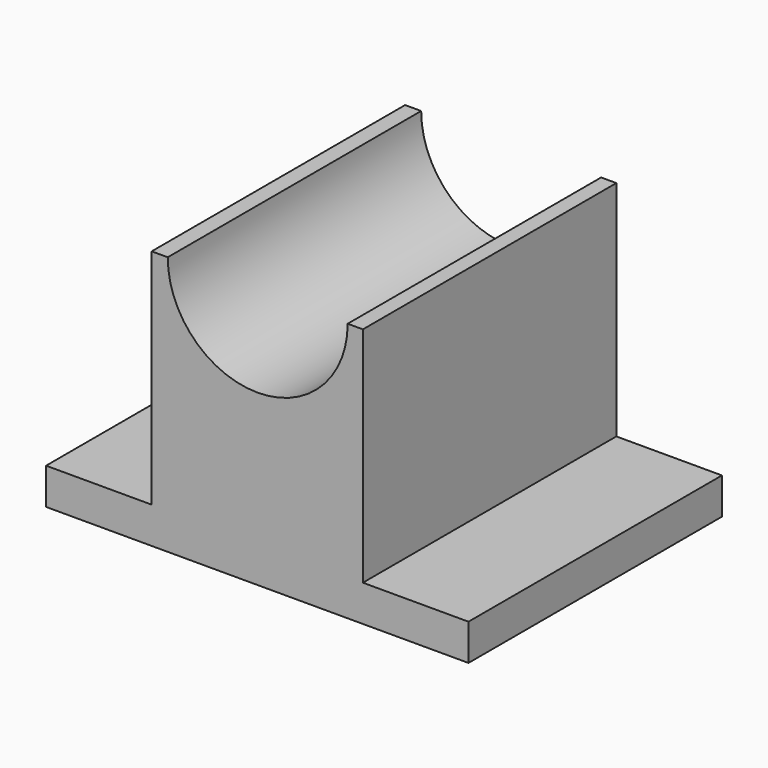
from build123d import *

# Parameters (mm, degrees)
F1_DEPTH = 114.3
F2_DEPTH = 114.3


# Not quite as in the source:
# - a feature names something its author has since deleted; it is built from what else it names


with BuildPart() as f1:
    # F0 (on Front) → F1 (new body)
    with BuildSketch(Plane.XZ):
        with BuildLine():
            Line((-32.3088020086, 46.7868000269), (-38.1029994101, 46.7868000269))
            Line((-38.1029994101, 46.7868000269), (-38.1029994101, -33.6804017425))
            Line((-38.1029994101, -33.6804017425), (-76.2000009418, -33.6804017425))
            Line((-76.2000009418, -33.6804017425), (-76.2000009418, -46.7868000269))
            Line((-76.2000009418, -46.7868000269), (-38.1029994101, -46.7868000269))
            Line((-38.1029994101, -46.7868000269), (38.1029994101, -46.7868000269))
            Line((38.1029994101, -46.7868000269), (76.2000009418, -46.7868000269))
            Line((76.2000009418, -46.7868000269), (76.2000009418, -33.6804017425))
            Line((76.2000009418, -33.6804017425), (38.1029994101, -33.6804017425))
            Line((38.1029994101, -33.6804017425), (38.1029994101, 46.7868000269))
            Line((38.1029994101, 46.7868000269), (32.6135978103, 46.7868000269))
            ThreePointArc((32.6135978103, 46.7868000269), (0.1523979008, 14.3256001174), (-32.3088020086, 46.7868000269))
        make_face()
    extrude(amount=F1_DEPTH)


with BuildPart() as f2:
    # F0 (on Front) → F2 (new body)
    with BuildSketch(Plane.XZ):
        with BuildLine():
            Line((-32.3088020086, 46.7868000269), (-38.1029994101, 46.7868000269))
            Line((-38.1029994101, 46.7868000269), (-38.1029994101, -33.6804017425))
            Line((-38.1029994101, -33.6804017425), (-76.2000009418, -33.6804017425))
            Line((-76.2000009418, -33.6804017425), (-76.2000009418, -46.7868000269))
            Line((-76.2000009418, -46.7868000269), (-38.1029994101, -46.7868000269))
            Line((-38.1029994101, -46.7868000269), (38.1029994101, -46.7868000269))
            Line((38.1029994101, -46.7868000269), (76.2000009418, -46.7868000269))
            Line((76.2000009418, -46.7868000269), (76.2000009418, -33.6804017425))
            Line((76.2000009418, -33.6804017425), (38.1029994101, -33.6804017425))
            Line((38.1029994101, -33.6804017425), (38.1029994101, 46.7868000269))
            Line((38.1029994101, 46.7868000269), (32.6135978103, 46.7868000269))
            ThreePointArc((32.6135978103, 46.7868000269), (0.1523979008, 14.3256001174), (-32.3088020086, 46.7868000269))
        make_face()
    extrude(amount=F2_DEPTH)


solid = Compound([f1.part, f2.part])
